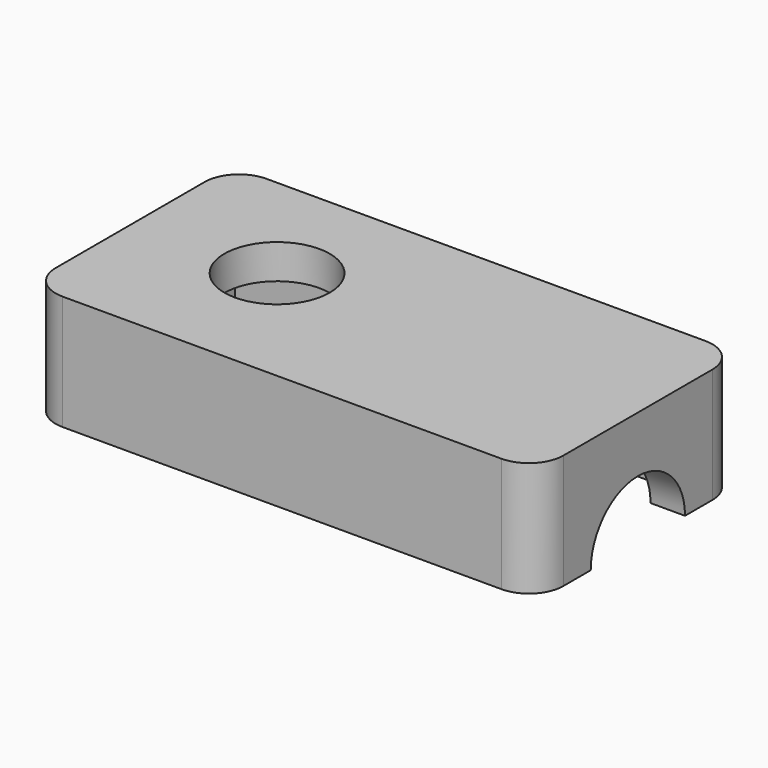
from build123d import *

# Parameters (mm, degrees)
F1_W         = 22.1
F1_H         = 11.1
F2_DEPTH     = 5
F0_W         = 19.1
F0_H         = 7.6
F3_DEPTH     = 3.5
F4_R         = 1.5
F5_R         = 2.2932815894
F6_DEPTH     = 4
F7_R         = 2.5647927057
F8_DEPTH     = 21
F9_TEXT_SIZE = 3.6068284923
F10_DEPTH    = 1


# Not quite as in the source:
# - Text() gives the source's letters only with a copy of the font that has no kerning and outlines rounded to 1/6400 em; it was checked with that copy


with BuildPart() as f2:
    # F1 (on Top) → F2 (new body)
    with BuildSketch(Plane.XY):
        with Locations((1.9605802372, -0.3473435954)):
            Rectangle(F1_W, F1_H)
    extrude(amount=F2_DEPTH)

    # F0 (on Top) → F3 (cut)
    with BuildSketch(Plane.XY):
        with Locations((1.9593628864, -0.3267633729)):
            Rectangle(F0_W, F0_H)
    extrude(amount=F3_DEPTH, mode=Mode.SUBTRACT)

    # F4
    f4_edges = [f2.edges().sort_by_distance(p)[0] for p in [
        (-9.08942, 5.202656, 2.5),
        (-9.08942, -5.897344, 2.5),
        (13.01058, 5.202656, 2.5),
        (13.01058, -5.897344, 2.5),
    ]]
    fillet(f4_edges, radius=F4_R)

    # F5 (on face) → F6 (cut)
    with BuildSketch(Plane.XY.offset(5)):
        with Locations((-2.9726461507, 0)):
            Circle(F5_R)
    extrude(amount=-F6_DEPTH, mode=Mode.SUBTRACT)

    # F7 (on face) → F8 (cut)
    with BuildSketch(Plane.YZ.offset(13.0105802372)):
        with Locations((-0.3473435954, 0)):
            Circle(F7_R)
    extrude(amount=-F8_DEPTH, mode=Mode.SUBTRACT)

    # F9 (on face) → F10 (cut)
    with BuildSketch(Plane(origin=(0, 0, 3.5), x_dir=(1, 0, 0), z_dir=(0, 0, -1))):
        with Locations((0.7287930348, -1.9013121491)):
            Text('rev02', F9_TEXT_SIZE, font='Open Sans', text_align=(TextAlign.LEFT, TextAlign.BOTTOM))
    extrude(amount=-F10_DEPTH, mode=Mode.SUBTRACT)


solid = f2.part
